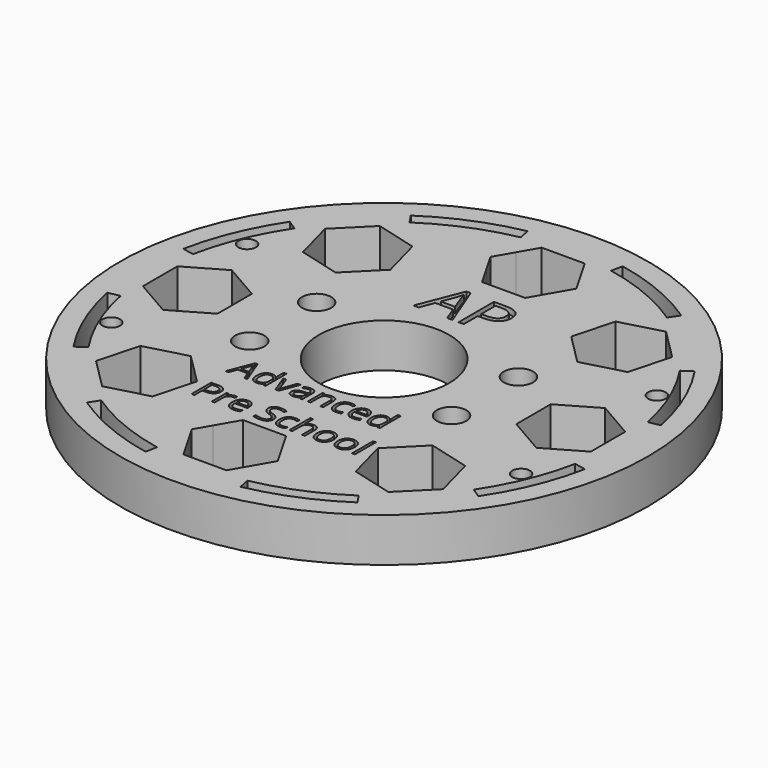
from build123d import *

# Parameters (mm, degrees)
F0_R           = 1.5
F0_R_2         = 2.5
F1_DEPTH       = 7.5
F2_TEXT_SIZE   = 10.5457820205
F2_TEXT_SIZE_2 = 5.8677991749
F3_DEPTH       = 1


# Not quite as in the source:
# - Text() gives the source's letters only with a copy of the font that has no kerning and outlines rounded to 1/6400 em; it was checked with that copy


with BuildPart() as f1:
    # F0 (on Top) → F1 (new body)
    with BuildSketch(Plane.XY):
        with BuildLine():
            ThreePointArc((0, -45), (31.8198051534, -31.8198051534), (45, 0))
            ThreePointArc((45, 0), (-31.8198051534, 31.8198051534), (0, -45))
        make_face()
        Polygon((-15.4216338358, -20.6063871247), (-16.5282228568, -24.7362335741), (-17.3193852519, -27.6888918297), (-18.7588436805, -28.0745935532), (-24.4018899569, -29.5866432458), (-29.5866432458, -24.4018899569), (-27.6888918297, -17.3193852519), (-20.6063871247, -15.4216338358), align=None, mode=Mode.SUBTRACT)
        with BuildLine():
            ThreePointArc((-21.9495327518, -32.8497972041), (-15.1191011199, -36.5007389747), (-7.707650911, -38.7489778163))
            Line((-7.707650911, -38.7489778163), (-8.0980722146, -40.7117582544))
            ThreePointArc((-8.0980722146, -40.7117582544), (-15.8849400554, -38.3496377192), (-23.0613585582, -34.5137621131))
            Line((-23.0613585582, -34.5137621131), (-21.9495327518, -32.8497972041))
        make_face(mode=Mode.SUBTRACT)
        with BuildLine():
            ThreePointArc((-38.7489778163, -7.707650911), (-36.5007389747, -15.1191011199), (-32.8497972041, -21.9495327518))
            Line((-32.8497972041, -21.9495327518), (-34.5137621131, -23.0613585582))
            ThreePointArc((-34.5137621131, -23.0613585582), (-38.3496377192, -15.8849400554), (-40.7117582544, -8.0980722146))
            Line((-40.7117582544, -8.0980722146), (-38.7489778163, -7.707650911))
        make_face(mode=Mode.SUBTRACT)
        with Locations((-34.9303736897, -14.468634521)):
            Circle(F0_R, mode=Mode.SUBTRACT)
        with Locations((-17.202949002, -7.1256947894)):
            Circle(F0_R_2, mode=Mode.SUBTRACT)
        with BuildLine():
            ThreePointArc((7.707650911, -38.7489778163), (15.1191011199, -36.5007389747), (21.9495327518, -32.8497972041))
            Line((21.9495327518, -32.8497972041), (23.0613585582, -34.5137621131))
            ThreePointArc((23.0613585582, -34.5137621131), (15.8849400554, -38.3496377192), (8.0980722146, -40.7117582544))
            Line((8.0980722146, -40.7117582544), (7.707650911, -38.7489778163))
        make_face(mode=Mode.SUBTRACT)
        Polygon((3.6661742094, -38.175657934), (0, -38.175657934), (-3.6661742094, -38.175657934), (-6.5872299068, -33.1162410542), (-7.3323484187, -31.825657934), (-5.8039400383, -29.1783769643), (-3.6661742094, -25.475657934), (0, -25.475657934), (3.6661742094, -25.475657934), (7.3323484187, -31.825657934), align=None, mode=Mode.SUBTRACT)
        Polygon((17.3193852519, -27.6888918297), (15.4216338358, -20.6063871247), (20.6063871247, -15.4216338358), (27.6888918297, -17.3193852519), (29.5866432458, -24.4018899569), (24.4018899569, -29.5866432458), align=None, mode=Mode.SUBTRACT)
        with Locations((17.202949002, -7.1256947894)):
            Circle(F0_R_2, mode=Mode.SUBTRACT)
        with Locations((34.9303736897, -14.468634521)):
            Circle(F0_R, mode=Mode.SUBTRACT)
        with BuildLine():
            ThreePointArc((32.8497972041, -21.9495327518), (36.5007389747, -15.1191011199), (38.7489778163, -7.707650911))
            Line((38.7489778163, -7.707650911), (40.7117582544, -8.0980722146))
            ThreePointArc((40.7117582544, -8.0980722146), (38.3496377192, -15.8849400554), (34.5137621131, -23.0613585582))
            Line((34.5137621131, -23.0613585582), (32.8497972041, -21.9495327518))
        make_face(mode=Mode.SUBTRACT)
        Polygon((31.825657934, -7.3323484187), (25.475657934, -3.6661742094), (25.475657934, 3.6661742094), (31.825657934, 7.3323484187), (38.175657934, 3.6661742094), (38.175657934, -3.6661742094), align=None, mode=Mode.SUBTRACT)
        Polygon((-31.825657934, 7.3323484187), (-25.475657934, 3.6661742094), (-25.475657934, -3.6661742094), (-31.825657934, -7.3323484187), (-38.175657934, -3.6661742094), (-38.175657934, 3.6661742094), align=None, mode=Mode.SUBTRACT)
        with BuildLine():
            ThreePointArc((-32.8497972041, 21.9495327518), (-36.5007389747, 15.1191011199), (-38.7489778163, 7.707650911))
            Line((-38.7489778163, 7.707650911), (-40.7117582544, 8.0980722146))
            ThreePointArc((-40.7117582544, 8.0980722146), (-38.3496377192, 15.8849400554), (-34.5137621131, 23.0613585582))
            Line((-34.5137621131, 23.0613585582), (-32.8497972041, 21.9495327518))
        make_face(mode=Mode.SUBTRACT)
        with Locations((-34.9303736897, 14.468634521)):
            Circle(F0_R, mode=Mode.SUBTRACT)
        with Locations((-17.202949002, 7.1256947894)):
            Circle(F0_R_2, mode=Mode.SUBTRACT)
        Polygon((-17.3193852519, 27.6888918297), (-15.4216338358, 20.6063871247), (-20.6063871247, 15.4216338358), (-27.6888918297, 17.3193852519), (-29.5866432458, 24.4018899569), (-24.4018899569, 29.5866432458), align=None, mode=Mode.SUBTRACT)
        with BuildLine():
            ThreePointArc((-7.707650911, 38.7489778163), (-15.1191011199, 36.5007389747), (-21.9495327518, 32.8497972041))
            Line((-21.9495327518, 32.8497972041), (-23.0613585582, 34.5137621131))
            ThreePointArc((-23.0613585582, 34.5137621131), (-15.8849400554, 38.3496377192), (-8.0980722146, 40.7117582544))
            Line((-8.0980722146, 40.7117582544), (-7.707650911, 38.7489778163))
        make_face(mode=Mode.SUBTRACT)
        with BuildLine():
            ThreePointArc((11.1125, 0), (7.8577241059, -7.8577241059), (0, -11.1125))
            ThreePointArc((0, -11.1125), (-1.0892154719, -11.0589902751), (-2.1679412034, -10.8989764285))
            ThreePointArc((-2.1679412034, -10.8989764285), (-4.2525696422, -10.266611305), (-6.1737742144, -9.2397060667))
            ThreePointArc((-6.1737742144, -9.2397060667), (-5.238396238, 9.8003500501), (11.1125, 0))
        make_face(mode=Mode.SUBTRACT)
        with Locations((17.202949002, 7.1256947894)):
            Circle(F0_R_2, mode=Mode.SUBTRACT)
        with Locations((34.9303736897, 14.468634521)):
            Circle(F0_R, mode=Mode.SUBTRACT)
        with BuildLine():
            ThreePointArc((38.7489778163, 7.707650911), (36.5007389747, 15.1191011199), (32.8497972041, 21.9495327518))
            Line((32.8497972041, 21.9495327518), (34.5137621131, 23.0613585582))
            ThreePointArc((34.5137621131, 23.0613585582), (38.3496377192, 15.8849400554), (40.7117582544, 8.0980722146))
            Line((40.7117582544, 8.0980722146), (38.7489778163, 7.707650911))
        make_face(mode=Mode.SUBTRACT)
        Polygon((3.6661742094, 38.175657934), (5.4992612729, 35.0006580052), (7.3323484187, 31.825657934), (5.4992613396, 28.6506579783), (3.6661742094, 25.475657934), (0, 25.475657934), (-3.6661742094, 25.475657934), (-5.4992613166, 28.6506579384), (-7.3323484187, 31.825657934), (-5.4992612741, 35.0006580032), (-3.6661742094, 38.175657934), (0, 38.175657934), align=None, mode=Mode.SUBTRACT)
        with BuildLine():
            ThreePointArc((21.9495327518, 32.8497972041), (15.1191011199, 36.5007389747), (7.707650911, 38.7489778163))
            Line((7.707650911, 38.7489778163), (8.0980722146, 40.7117582544))
            ThreePointArc((8.0980722146, 40.7117582544), (15.8849400554, 38.3496377192), (23.0613585582, 34.5137621131))
            Line((23.0613585582, 34.5137621131), (21.9495327518, 32.8497972041))
        make_face(mode=Mode.SUBTRACT)
        Polygon((27.6888918297, 17.3193852519), (20.6063871247, 15.4216338358), (15.4216338358, 20.6063871247), (17.3193852519, 27.6888918297), (24.4018899569, 29.5866432458), (29.5866432458, 24.4018899569), align=None, mode=Mode.SUBTRACT)
    extrude(amount=F1_DEPTH)

    # F2 (on face) → F3 (cut)
    with BuildSketch(Plane.XY.offset(7.5)):
        with Locations((-6.5828748706, 14.4753102213)):
            Text('AP', F2_TEXT_SIZE, font='Open Sans', text_align=(TextAlign.LEFT, TextAlign.BOTTOM))
        with Locations((-14.2866559327, -15.9104978666)):
            Text('Advanced', F2_TEXT_SIZE_2, font='Open Sans', text_align=(TextAlign.LEFT, TextAlign.BOTTOM))
        with Locations((-14.2866559327, -23.8907047444)):
            Text('Pre School', F2_TEXT_SIZE_2, font='Open Sans', text_align=(TextAlign.LEFT, TextAlign.BOTTOM))
    extrude(amount=-F3_DEPTH, mode=Mode.SUBTRACT)


solid = f1.part
